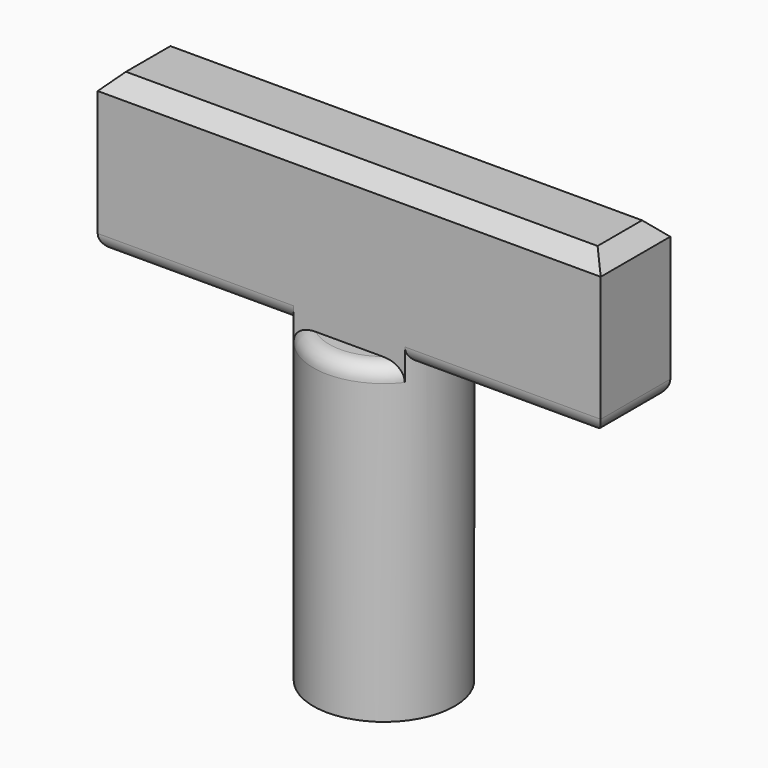
from build123d import *

# Parameters (mm, degrees)
F0_R        = 4.5
F1_DEPTH    = 20
F2_W        = 7.0876832783
F2_H        = 5.546597673
F3_DEPTH    = 10
F4_DEPTH    = 12.5
F5_SIZE     = 1
F6_T4_ANGLE = 167.6048406122
F6_T9_ANGLE = 167.6048406122
F7_R        = 1


# Not quite as in the source:
# - a fillet or chamfer that OpenCascade refuses, or shapes differently, is made with other operations: its cross-section is extruded or revolved along the edge and cut away or added


with BuildPart() as f1:
    # F0 (on Top) → F1 (new body)
    with BuildSketch(Plane.XY):
        Circle(F0_R)
        with BuildLine():
            ThreePointArc((2.2, 1.1874342087), (2.4238399287, 0.6123724357), (2.5, 0))
            ThreePointArc((2.5, 0), (2.4238399287, -0.6123724357), (2.2, -1.1874342087))
            ThreePointArc((2.2, -1.1874342087), (-2.5, 0), (2.2, 1.1874342087))
        make_face(mode=Mode.SUBTRACT)
        with BuildLine():
            ThreePointArc((2.2, -1.1874342087), (2.4238399287, -0.6123724357), (2.5, 0))
            ThreePointArc((2.5, 0), (2.4238399287, 0.6123724357), (2.2, 1.1874342087))
            Line((2.2, 1.1874342087), (2.2, -1.1874342087))
        make_face()
    extrude(amount=F1_DEPTH)

    # F2 (on face) → F3 (join)
    with BuildSketch(Plane.XY.offset(20)):
        Rectangle(F2_W, F2_H)
        with BuildLine():
            Line((2.2, 1.1874342087), (2.2, -1.1874342087))
            ThreePointArc((2.2, -1.1874342087), (-2.5, 0), (2.2, 1.1874342087))
        make_face(mode=Mode.SUBTRACT)
    extrude(amount=F3_DEPTH)

    # F4 (add, symmetric): faces of the model
    f4_faces = [f1.faces().sort_by_distance(p)[0] for p in [
        (3.5438416392, 0, 25),
        (-3.5438416392, 0, 25),
    ]]
    extrude(f4_faces, amount=F4_DEPTH, both=True, dir=(1, 0, 0))

    # F5
    f5_edges = [f1.edges().sort_by_distance(p)[0] for p in [
        (0, -2.773299, 30),
        (0, 2.773299, 30),
        (16.043842, 0, 30),
        (-16.043842, 0, 30),
    ]]
    chamfer(f5_edges, length=F5_SIZE)

    # F6: fillet of radius 1 on 2 edges, made by hand


with BuildPart() as f6_tool2:
    # F6_s3 → F6_t4 (revolve)
    with BuildSketch(Plane(origin=(0, 0, 0), x_dir=(0, 0, 1), z_dir=(0.1079573604, -0.9941555252, 0))):
        with BuildLine():
            ThreePointArc((20, -3.5), (19.7071067812, -4.2071067812), (19, -4.5))
            Line((19, -4.5), (20, -4.5))
            Line((20, -4.5), (20, -3.5))
        make_face()
    revolve(axis=Axis((0, 0, 20), (0, 0, 1)), revolution_arc=F6_T4_ANGLE)

    split(bisect_by=Plane.XZ.offset(-2.7732988365), keep=Keep.BOTTOM)


with BuildPart() as f1_1:
    add(f1.part)

    # F6_t1: cut F6_tool2
    add(f6_tool2.part, mode=Mode.SUBTRACT)


with BuildPart() as f6_tool7:
    # F6_s8 → F6_t9 (revolve)
    with BuildSketch(Plane(origin=(0, 0, 0), x_dir=(0, 0, 1), z_dir=(-0.1079573604, 0.9941555252, 0))):
        with BuildLine():
            ThreePointArc((19, -4.5), (19.7071067812, -4.2071067812), (20, -3.5))
            Line((20, -3.5), (20, -4.5))
            Line((20, -4.5), (19, -4.5))
        make_face()
    revolve(axis=Axis((0, 0, 20), (0, 0, 1)), revolution_arc=F6_T9_ANGLE)

    split(bisect_by=Plane.XZ.offset(2.7732988365), keep=Keep.TOP)


with BuildPart() as f1_2:
    add(f1_1.part)

    # F6_t6: cut F6_tool7
    add(f6_tool7.part, mode=Mode.SUBTRACT)

    # F7
    f7_edges = [f1_2.edges().sort_by_distance(p)[0] for p in [
        (9.793842, 2.773299, 20),
        (-9.793842, 2.773299, 20),
        (9.793842, -2.773299, 20),
        (-9.793842, -2.773299, 20),
        (16.043842, 0, 20),
        (-16.043842, 0, 20),
    ]]
    fillet(f7_edges, radius=F7_R)


solid = f1_2.part
